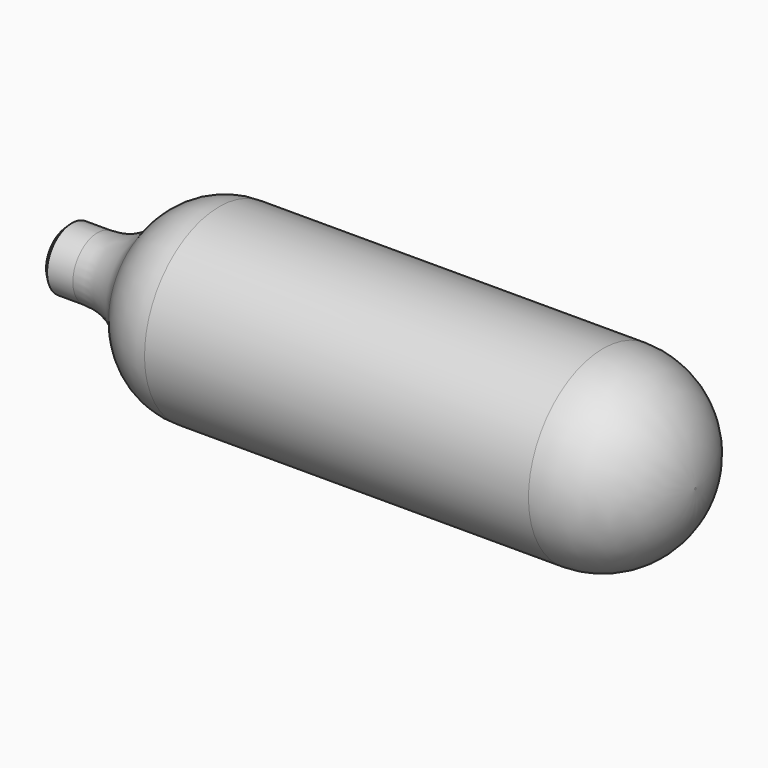
from build123d import *

# Parameters (mm, degrees)
F2_R    = 9.398
F4_R    = 7.62
F5_SIZE = 0.508


# Not quite as in the source:
# - a fillet or chamfer that OpenCascade refuses, or shapes differently, is made with other operations: its cross-section is extruded or revolved along the edge and cut away or added


with BuildPart() as f1:
    # F0 (on Front) → F1 (revolve)
    with BuildSketch(Plane.XZ):
        Polygon((0, 3.1496), (0, 0), (64.008, 0), (64.008, 9.4996), (8.001, 9.4996), (8.001, 3.1496), align=None)
    revolve(axis=Axis((-4.5283841901, 0, 0), (-1, 0, 0)))

    # F2
    f2_edges = [f1.edges().sort_by_distance(p)[0] for p in [
        (64.008, 0, -9.4996),
    ]]
    fillet(f2_edges, radius=F2_R)

    # F3: fillet of radius 7.62 on 1 edges, made by hand

    # F3_s1 → F3_t2 (revolve, cut)
    with BuildSketch(Plane.XZ):
        with BuildLine():
            ThreePointArc((15.5144213245, 9.4996), (10.5957324749, 7.6994711326), (8.001, 3.1496))
            Line((8.001, 3.1496), (8.001, 9.4996))
            Line((8.001, 9.4996), (15.5144213245, 9.4996))
        make_face()
    revolve(axis=Axis((8.001, 0, 0), (-1, 0, 0)), mode=Mode.SUBTRACT)

    # F4
    f4_edges = [f1.edges().sort_by_distance(p)[0] for p in [
        (8.001, 0, -3.1496),
    ]]
    fillet(f4_edges, radius=F4_R)

    # F5
    f5_edges = [f1.edges().sort_by_distance(p)[0] for p in [
        (0, 0, -3.1496),
    ]]
    chamfer(f5_edges, length=F5_SIZE)


solid = f1.part
